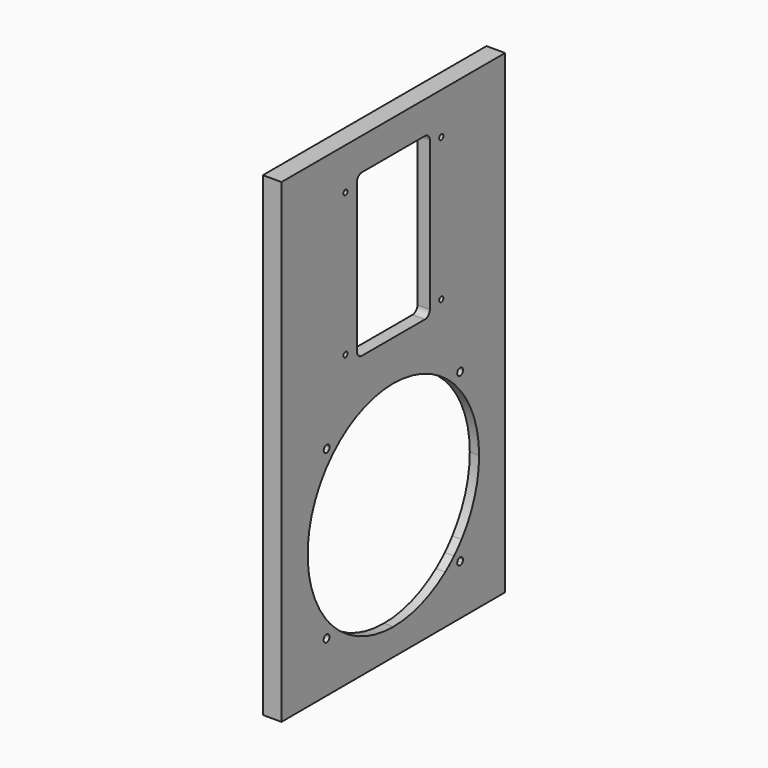
from build123d import *

# Parameters (mm, degrees)
F1_DEPTH = 9
F2_R     = 9
F3_DEPTH = 4.5
F4_DEPTH = 6


# Not quite as in the source:
# - ends of sketch curves that miss each other by under 0.0002 mm in the source are joined


with BuildPart() as f1:
    # F0 (on Right) → F1 (new body)
    with BuildSketch(Plane.YZ):
        Polygon((68.1698566968, 98.8894649375), (-66.8301433032, 98.8894649375), (-66.8301433032, -130.6578782697), (-12.3170643615, -130.5693798602), (0.7047325379, -130.5482398267), (13.9946170468, -130.5266645706), (68.1698566968, -130.438714621), align=None)
        with BuildLine():
            ThreePointArc((48.4358981994, -113.62957348), (25.065280219, -120.9302143017), (0.7053488138, -123.3957534174))
            ThreePointArc((0.7053488138, -123.3957534174), (-23.6541573557, -120.9260165144), (-47.0235169065, -113.6213484606))
            ThreePointArc((-47.0235169065, -113.6213484606), (-54.3241821931, -90.2506109118), (-56.7896968225, -65.8905549838))
            ThreePointArc((-56.7896968225, -65.8905549838), (-54.3199354552, -41.5311733414), (-47.015291887, -18.1619333547))
            ThreePointArc((-47.015291887, -18.1619333547), (-23.6446739066, -10.861292533), (0.7152574986, -8.3957534174))
            ThreePointArc((0.7152574986, -8.3957534174), (25.0747636681, -10.8654903203), (48.4441232188, -18.1701583742))
            ThreePointArc((48.4441232188, -18.1701583742), (58.2103031562, -65.9007077597), (48.4358981994, -113.62957348))
        make_face(mode=Mode.SUBTRACT)
        with BuildLine():
            add(Edge.make_bspline(
                [(29.3361078756, 2.5166290842), (19.796011102, -0.2153058112), (10.2559143284, -1.8939046488), (0.7158175548, -1.8957518912)],
                knots=[0.0757162728, 0.0757162728, 0.0757162728, 0.0757162728, 0.4997664403, 0.4997664403, 0.4997664403, 0.4997664403], degree=3))
            add(Edge.make_bspline(
                [(0.7158175548, -1.8957518912), (0.7105630297, -1.8957529086), (-8.8393481458, -1.8966775746), (-18.3892593212, -0.2170548711), (-27.9339159716, 2.5160323353)],
                knots=[0.4997664403, 0.4997664403, 0.4997664403, 0.4997664403, 0.5, 0.9242528506, 0.9242528506, 0.9242528506, 0.9242528506], degree=3))
            add(Edge.make_bspline(
                [(-27.9339159716, 2.5160323353), (-29.5600423042, 2.981669313), (-31.1861686369, 3.477911029), (-32.8122949696, 4.0016701601)],
                knots=[0.9242528506, 0.9242528506, 0.9242528506, 0.9242528506, 0.99653295, 0.99653295, 0.99653295, 0.99653295], degree=3))
            add(Edge.make_bspline(
                [(-32.8122949696, 4.0016701601), (-32.890295156, 4.026793245), (-32.9682953425, 4.0519796425), (-33.046295529, 4.0772290119)],
                knots=[0.99653295, 0.99653295, 0.99653295, 0.99653295, 1, 1, 1, 1], degree=3))
            add(Edge.make_bspline(
                [(-33.046295529, 4.0772290119), (-33.6603555303, 5.82974856), (-34.2037564934, 7.5898287802), (-34.6844360116, 9.3555033957)],
                knots=[0, 0, 0, 0, 0.0653643369, 0.0653643369, 0.0653643369, 0.0653643369], degree=3))
            add(Edge.make_bspline(
                [(-34.6844360116, 9.3555033957), (-37.9202250753, 21.2414906157), (-38.6995984681, 45.2840048827), (-37.8280446873, 67.9681639939), (-34.6344472565, 79.4497202748)],
                knots=[0.0653643369, 0.0653643369, 0.0653643369, 0.0653643369, 0.505377274, 0.9368183556, 0.9368183556, 0.9368183556, 0.9368183556], degree=3))
            add(Edge.make_bspline(
                [(-34.6344472565, 79.4497202748), (-34.166766394, 81.1311169635), (-33.6398504009, 82.8178973737), (-33.046295529, 84.5118955394)],
                knots=[0.9368183556, 0.9368183556, 0.9368183556, 0.9368183556, 1, 1, 1, 1], degree=3))
            add(Edge.make_bspline(
                [(-33.046295529, 84.5118955394), (-31.407102949, 85.0425170785), (-29.767910369, 85.5461701309), (-28.128717789, 86.0194468275)],
                knots=[0, 0, 0, 0, 0.0728608844, 0.0728608844, 0.0728608844, 0.0728608844], degree=3))
            add(Edge.make_bspline(
                [(-28.128717789, 86.0194468275), (-18.5191271995, 88.7939806713), (-8.9045783182, 90.52544354), (0.7099705632, 90.5245501515), (0.714928855, 90.5245492301)],
                knots=[0.0728608844, 0.0728608844, 0.0728608844, 0.0728608844, 0.5, 0.5002203924, 0.5002203924, 0.5002203924, 0.5002203924], degree=3))
            add(Edge.make_bspline(
                [(0.714928855, 90.5245492301), (10.3175892534, 90.5227648451), (19.9202496517, 88.7932594642), (29.52291005, 86.0211547084)],
                knots=[0.5002203924, 0.5002203924, 0.5002203924, 0.5002203924, 0.9270514662, 0.9270514662, 0.9270514662, 0.9270514662], degree=3))
            add(Edge.make_bspline(
                [(29.52291005, 86.0211547084), (31.1640745294, 85.5473818508), (32.8052390087, 85.0431554002), (34.4464034881, 84.5118955394)],
                knots=[0.9270514662, 0.9270514662, 0.9270514662, 0.9270514662, 1, 1, 1, 1], degree=3))
            add(Edge.make_bspline(
                [(34.4464034881, 84.5118955394), (35.0441587431, 82.8122899736), (35.5738699066, 81.1245502388), (36.0432502856, 79.4456408795)],
                knots=[0, 0, 0, 0, 0.0633907856, 0.0633907856, 0.0633907856, 0.0633907856], degree=3))
            add(Edge.make_bspline(
                [(36.0432502856, 79.4456408795), (39.2115398843, 68.1131027115), (40.0658474487, 45.8547250069), (39.3582763009, 21.3935099545), (36.0875285415, 9.3598851242)],
                knots=[0.0633907856, 0.0633907856, 0.0633907856, 0.0633907856, 0.4912748121, 0.9347375535, 0.9347375535, 0.9347375535, 0.9347375535], degree=3))
            add(Edge.make_bspline(
                [(36.0875285415, 9.3598851242), (35.6061870876, 7.5889498832), (35.0618079197, 5.8270167192), (34.4464034881, 4.0772290119)],
                knots=[0.9347375535, 0.9347375535, 0.9347375535, 0.9347375535, 1, 1, 1, 1], degree=3))
            add(Edge.make_bspline(
                [(34.4464034881, 4.0772290119), (34.3822403491, 4.0564588206), (34.3180772102, 4.0357312407), (34.2539140712, 4.015046462)],
                knots=[0, 0, 0, 0, 0.0028520035, 0.0028520035, 0.0028520035, 0.0028520035], degree=3))
            add(Edge.make_bspline(
                [(34.2539140712, 4.015046462), (32.6146453394, 3.4865824325), (30.9753766075, 2.9860557114), (29.3361078756, 2.5166290842)],
                knots=[0.0028520035, 0.0028520035, 0.0028520035, 0.0028520035, 0.0757162728, 0.0757162728, 0.0757162728, 0.0757162728], degree=3))
        make_face(mode=Mode.SUBTRACT)
        with BuildLine():
            ThreePointArc((33.489766199, 4.9329490876), (31.5635091045, 3.4659554383), (29.3361078756, 2.5166290842))
            add(Edge.make_bspline(
                [(34.2539140712, 4.015046462), (32.6146453394, 3.4865824325), (30.9753766075, 2.9860557114), (29.3361078756, 2.5166290842)],
                knots=[0.0028520035, 0.0028520035, 0.0028520035, 0.0028520035, 0.0757162728, 0.0757162728, 0.0757162728, 0.0757162728], degree=3))
            Line((34.2539140712, 4.015046462), (33.489766199, 4.9329490876))
        make_face()
        with BuildLine():
            add(Edge.make_bspline(
                [(-27.9339159716, 2.5160323353), (-29.5600423042, 2.981669313), (-31.1861686369, 3.477911029), (-32.8122949696, 4.0016701601)],
                knots=[0.9242528506, 0.9242528506, 0.9242528506, 0.9242528506, 0.99653295, 0.99653295, 0.99653295, 0.99653295], degree=3))
            ThreePointArc((-27.9339159716, 2.5160323353), (-30.1447439704, 3.4556982526), (-32.0601500824, 4.9055092414))
            Line((-32.0601500824, 4.9055092414), (-32.8122949696, 4.0016701601))
        make_face()
        with BuildLine():
            Line((33.489766199, 4.9329490876), (34.2539140712, 4.015046462))
            add(Edge.make_bspline(
                [(34.4464034881, 4.0772290119), (34.3822403491, 4.0564588206), (34.3180772102, 4.0357312407), (34.2539140712, 4.015046462)],
                knots=[0, 0, 0, 0, 0.0028520035, 0.0028520035, 0.0028520035, 0.0028520035], degree=3))
            add(Edge.make_bspline(
                [(36.0875285415, 9.3598851242), (35.6061870876, 7.5889498832), (35.0618079197, 5.8270167192), (34.4464034881, 4.0772290119)],
                knots=[0.9347375535, 0.9347375535, 0.9347375535, 0.9347375535, 1, 1, 1, 1], degree=3))
            ThreePointArc((36.0875285415, 9.3598851242), (35.0839686926, 6.9731201339), (33.489766199, 4.9329490876))
        make_face()
        with BuildLine():
            add(Edge.make_bspline(
                [(-32.8122949696, 4.0016701601), (-32.890295156, 4.026793245), (-32.9682953425, 4.0519796425), (-33.046295529, 4.0772290119)],
                knots=[0.99653295, 0.99653295, 0.99653295, 0.99653295, 1, 1, 1, 1], degree=3))
            Line((-32.8122949696, 4.0016701601), (-32.0601500824, 4.9055092414))
            ThreePointArc((-32.0601500824, 4.9055092414), (-33.6711503863, 6.9542617926), (-34.6844360116, 9.3555033957))
            add(Edge.make_bspline(
                [(-33.046295529, 4.0772290119), (-33.6603555303, 5.82974856), (-34.2037564934, 7.5898287802), (-34.6844360116, 9.3555033957)],
                knots=[0, 0, 0, 0, 0.0653643369, 0.0653643369, 0.0653643369, 0.0653643369], degree=3))
        make_face()
        with BuildLine():
            ThreePointArc((29.52291005, 86.0211547084), (33.6376071248, 83.5807546158), (36.0432502856, 79.4456408795))
            add(Edge.make_bspline(
                [(34.4464034881, 84.5118955394), (35.0441587431, 82.8122899736), (35.5738699066, 81.1245502388), (36.0432502856, 79.4456408795)],
                knots=[0, 0, 0, 0, 0.0633907856, 0.0633907856, 0.0633907856, 0.0633907856], degree=3))
            add(Edge.make_bspline(
                [(29.52291005, 86.0211547084), (31.1640745294, 85.5473818508), (32.8052390087, 85.0431554002), (34.4464034881, 84.5118955394)],
                knots=[0.9270514662, 0.9270514662, 0.9270514662, 0.9270514662, 1, 1, 1, 1], degree=3))
        make_face()
        with BuildLine():
            add(Edge.make_bspline(
                [(-34.6344472565, 79.4497202748), (-34.166766394, 81.1311169635), (-33.6398504009, 82.8178973737), (-33.046295529, 84.5118955394)],
                knots=[0.9368183556, 0.9368183556, 0.9368183556, 0.9368183556, 1, 1, 1, 1], degree=3))
            ThreePointArc((-34.6344472565, 79.4497202748), (-32.2364800237, 83.5811533161), (-28.128717789, 86.0194468275))
            add(Edge.make_bspline(
                [(-33.046295529, 84.5118955394), (-31.407102949, 85.0425170785), (-29.767910369, 85.5461701309), (-28.128717789, 86.0194468275)],
                knots=[0, 0, 0, 0, 0.0728608844, 0.0728608844, 0.0728608844, 0.0728608844], degree=3))
        make_face()
    extrude(amount=-F1_DEPTH)

    # F2
    f2_edges = [f1.edges().sort_by_distance(p)[0] for p in [
        (-4.5, 48.444123, -18.170158),
        (-4.5, -47.015292, -18.161933),
        (-4.5, 48.435898, -113.629573),
        (-4.5, -47.023517, -113.621348),
    ]]
    fillet(f2_edges, radius=F2_R)

    # F0 (on Right) → F3 (join)
    with BuildSketch(Plane.YZ):
        with BuildLine():
            ThreePointArc((-47.0235169065, -113.6213484606), (-23.6541573557, -120.9260165144), (0.7053488138, -123.3957534174))
            Line((0.7053488138, -123.3957534174), (0.7058442481, -117.6457532253))
            ThreePointArc((0.7058442481, -117.6457532253), (-15.8462466549, -114.9257764477), (-30.6588276682, -107.0544721939))
            ThreePointArc((-30.6588276682, -107.0544721939), (-37.7060174416, -114.9920661148), (-47.4126185448, -110.6966993112))
            ThreePointArc((-47.4126185448, -110.6966993112), (-48.2050884281, -108.8920718604), (-48.5857259237, -106.9582146141))
            add(Edge.make_bspline(
                [(-48.5857259237, -106.9582146141), (-52.8599458618, -93.2689444024), (-56.7908900644, -79.5796204898), (-56.7896968298, -65.8906363475), (-56.7896968225, -65.8905549838)],
                knots=[0.0417183372, 0.0417183372, 0.0417183372, 0.0417183372, 0.5000000605, 0.5000027845, 0.5000027845, 0.5000027845, 0.5000027845], degree=3))
            ThreePointArc((-56.7896968225, -65.8905549838), (-54.3241821931, -90.2506109118), (-47.0235169065, -113.6213484606))
        make_face()
        with BuildLine():
            Line((0.7058442481, -117.6457532253), (0.7053488138, -123.3957534174))
            ThreePointArc((0.7053488138, -123.3957534174), (25.065280219, -120.9302143017), (48.4358981994, -113.62957348))
            ThreePointArc((48.4358981994, -113.62957348), (58.2103031562, -65.9007077597), (48.4441232188, -18.1701583742))
            Line((48.4441232188, -18.1701583742), (42.246463418, -24.3667502557))
            ThreePointArc((42.246463418, -24.3667502557), (42.6184588324, -24.9309450129), (42.7489434931, -25.594021227))
            ThreePointArc((42.7489434931, -25.594021227), (41.6751090125, -27.2081154593), (39.7714575612, -26.8413296439))
            Line((39.7714575612, -26.8413296439), (37.3062318709, -29.3061305509))
            ThreePointArc((37.3062318709, -29.3061305509), (48.5219220944, -46.0939455578), (52.4603031562, -65.8957534174))
            ThreePointArc((52.4603031562, -65.8957534174), (49.7443824638, -82.4402862442), (41.8816918922, -97.2482533105))
            ThreePointArc((41.8816918922, -97.2482533105), (47.6632613149, -100.162881038), (49.9922390805, -106.2041940035))
            ThreePointArc((49.9922390805, -106.2041940035), (49.3222308171, -109.6117206236), (47.4119640434, -112.5118981342))
            ThreePointArc((47.4119640434, -112.5118981342), (37.9982171595, -114.6915865794), (32.0357152763, -107.0877557419))
            ThreePointArc((32.0357152763, -107.0877557419), (17.2365960025, -114.9359832777), (0.7058442481, -117.6457532253))
        make_face()
        with BuildLine():
            ThreePointArc((-47.4126185448, -110.6966993112), (-37.7060174416, -114.9920661148), (-30.6588276682, -107.0544721939))
            ThreePointArc((-30.6588276682, -107.0544721939), (-33.3488280366, -104.8577616098), (-35.8854305819, -102.4855712929))
            ThreePointArc((-35.8854305819, -102.4855712929), (-38.2656491214, -99.9389266546), (-40.4690269301, -97.2378221691))
            ThreePointArc((-40.4690269301, -97.2378221691), (-46.5261994153, -100.4289659711), (-48.5857259237, -106.9582146141))
            add(Edge.make_bspline(
                [(-47.4126185448, -110.6966993112), (-47.8046988201, -109.4505402503), (-48.1966348041, -108.2043773175), (-48.5857259237, -106.9582146141)],
                knots=[0, 0, 0, 0, 0.0417183372, 0.0417183372, 0.0417183372, 0.0417183372], degree=3))
        make_face()
        with BuildLine():
            ThreePointArc((-40.8454512075, -107.4447669293), (-40.8552676402, -104.9599498094), (-38.3704521876, -104.9701795704))
            ThreePointArc((-38.3704521876, -104.9701795704), (-37.9984287346, -105.5343880299), (-37.867933696, -106.1974895908))
            ThreePointArc((-37.867933696, -106.1974895908), (-38.9417886099, -107.8115923826), (-40.8454512075, -107.4447669293))
        make_face(mode=Mode.SUBTRACT)
        with BuildLine():
            ThreePointArc((37.3466484089, -102.4449080796), (34.7703842615, -104.8569312114), (32.0357152763, -107.0877557419))
            ThreePointArc((32.0357152763, -107.0877557419), (37.9982171595, -114.6915865794), (47.4119640434, -112.5118981342))
            Line((47.4119640434, -112.5118981342), (42.284825174, -107.3839063374))
            ThreePointArc((42.284825174, -107.3839063374), (39.754699299, -107.4415279477), (39.8127417737, -104.9114116926))
            Line((39.8127417737, -104.9114116926), (37.3466484089, -102.4449080796))
        make_face()
        with BuildLine():
            ThreePointArc((-47.015291887, -18.1619333547), (-54.3199354552, -41.5311733414), (-56.7896968225, -65.8905549838))
            add(Edge.make_bspline(
                [(-48.5857259237, -106.9582146141), (-52.8599458618, -93.2689444024), (-56.7908900644, -79.5796204898), (-56.7896968298, -65.8906363475), (-56.7896968225, -65.8905549838)],
                knots=[0.0417183372, 0.0417183372, 0.0417183372, 0.0417183372, 0.5000000605, 0.5000027845, 0.5000027845, 0.5000027845, 0.5000027845], degree=3))
            ThreePointArc((-48.5857259237, -106.9582146141), (-46.5261994153, -100.4289659711), (-40.4690269301, -97.2378221691))
            ThreePointArc((-40.4690269301, -97.2378221691), (-50.9220063581, -62.4076143407), (-35.8793197103, -29.2998247027))
            Line((-35.8793197103, -29.2998247027), (-38.353980194, -26.8247377365))
            ThreePointArc((-38.353980194, -26.8247377365), (-40.8288539189, -26.8245244952), (-40.8286406777, -24.3496507703))
            Line((-40.8286406777, -24.3496507703), (-45.9547231085, -19.2226849115))
            Line((-45.9547231085, -19.2226849115), (-47.015291887, -18.1619333547))
        make_face()
        with BuildLine():
            Line((42.246463418, -24.3667502557), (48.4441232188, -18.1701583742))
            ThreePointArc((48.4441232188, -18.1701583742), (25.0747636681, -10.8654903203), (0.7152574986, -8.3957534174))
            Line((0.7152574986, -8.3957534174), (0.7147620643, -14.1457536095))
            ThreePointArc((0.7147620643, -14.1457536095), (20.5182902015, -18.0866941376), (37.3062318709, -29.3061305509))
            Line((37.3062318709, -29.3061305509), (39.7714575612, -26.8413296439))
            ThreePointArc((39.7714575612, -26.8413296439), (39.7616132513, -24.3564777439), (42.246463418, -24.3667502557))
        make_face()
        with BuildLine():
            ThreePointArc((-48.5857259237, -106.9582146141), (-48.2050884281, -108.8920718604), (-47.4126185448, -110.6966993112))
            add(Edge.make_bspline(
                [(-47.4126185448, -110.6966993112), (-47.8046988201, -109.4505402503), (-48.1966348041, -108.2043773175), (-48.5857259237, -106.9582146141)],
                knots=[0, 0, 0, 0, 0.0417183372, 0.0417183372, 0.0417183372, 0.0417183372], degree=3))
        make_face()
        with BuildLine():
            ThreePointArc((41.8816918922, -97.2482533105), (39.7008426794, -99.9222185246), (37.3466484089, -102.4449080796))
            Line((37.3466484089, -102.4449080796), (39.8127417737, -104.9114116926))
            ThreePointArc((39.8127417737, -104.9114116926), (41.6987727715, -104.6031599179), (42.7422390805, -106.2041940035))
            ThreePointArc((42.7422390805, -106.2041940035), (42.6238832916, -106.8368370056), (42.284825174, -107.3839063374))
            Line((42.284825174, -107.3839063374), (47.4119640434, -112.5118981342))
            ThreePointArc((47.4119640434, -112.5118981342), (49.3222308171, -109.6117206236), (49.9922390805, -106.2041940035))
            ThreePointArc((49.9922390805, -106.2041940035), (47.6632613149, -100.162881038), (41.8816918922, -97.2482533105))
        make_face()
        with BuildLine():
            ThreePointArc((0.7152574986, -8.3957534174), (-23.6446739066, -10.861292533), (-47.015291887, -18.1619333547))
            Line((-47.015291887, -18.1619333547), (-45.9547231085, -19.2226849115))
            Line((-45.9547231085, -19.2226849115), (-40.8286406777, -24.3496507703))
            ThreePointArc((-40.8286406777, -24.3496507703), (-38.9215447765, -23.9704339243), (-37.8413104358, -25.5871942534))
            ThreePointArc((-37.8413104358, -25.5871942534), (-37.9745501068, -26.2569599127), (-38.353980194, -26.8247377365))
            Line((-38.353980194, -26.8247377365), (-35.8793197103, -29.2998247027))
            ThreePointArc((-35.8793197103, -29.2998247027), (-19.0894449013, -18.0832814371), (0.7147620643, -14.1457536095))
            Line((0.7147620643, -14.1457536095), (0.7152574986, -8.3957534174))
        make_face()
        with BuildLine():
            ThreePointArc((33.489766199, 4.9329490876), (31.5635091045, 3.4659554383), (29.3361078756, 2.5166290842))
            add(Edge.make_bspline(
                [(34.2539140712, 4.015046462), (32.6146453394, 3.4865824325), (30.9753766075, 2.9860557114), (29.3361078756, 2.5166290842)],
                knots=[0.0028520035, 0.0028520035, 0.0028520035, 0.0028520035, 0.0757162728, 0.0757162728, 0.0757162728, 0.0757162728], degree=3))
            Line((34.2539140712, 4.015046462), (33.489766199, 4.9329490876))
        make_face()
        with BuildLine():
            add(Edge.make_bspline(
                [(-27.9339159716, 2.5160323353), (-29.5600423042, 2.981669313), (-31.1861686369, 3.477911029), (-32.8122949696, 4.0016701601)],
                knots=[0.9242528506, 0.9242528506, 0.9242528506, 0.9242528506, 0.99653295, 0.99653295, 0.99653295, 0.99653295], degree=3))
            ThreePointArc((-27.9339159716, 2.5160323353), (-30.1447439704, 3.4556982526), (-32.0601500824, 4.9055092414))
            Line((-32.0601500824, 4.9055092414), (-32.8122949696, 4.0016701601))
        make_face()
        with BuildLine():
            Line((33.489766199, 4.9329490876), (34.2539140712, 4.015046462))
            add(Edge.make_bspline(
                [(34.4464034881, 4.0772290119), (34.3822403491, 4.0564588206), (34.3180772102, 4.0357312407), (34.2539140712, 4.015046462)],
                knots=[0, 0, 0, 0, 0.0028520035, 0.0028520035, 0.0028520035, 0.0028520035], degree=3))
            add(Edge.make_bspline(
                [(36.0875285415, 9.3598851242), (35.6061870876, 7.5889498832), (35.0618079197, 5.8270167192), (34.4464034881, 4.0772290119)],
                knots=[0.9347375535, 0.9347375535, 0.9347375535, 0.9347375535, 1, 1, 1, 1], degree=3))
            ThreePointArc((36.0875285415, 9.3598851242), (35.0839686926, 6.9731201339), (33.489766199, 4.9329490876))
        make_face()
        with BuildLine():
            Line((30.2969391288, 8.7682072326), (33.489766199, 4.9329490876))
            ThreePointArc((33.489766199, 4.9329490876), (35.0839686926, 6.9731201339), (36.0875285415, 9.3598851242))
            add(Edge.make_bspline(
                [(36.0432502856, 79.4456408795), (39.2115398843, 68.1131027115), (40.0658474487, 45.8547250069), (39.3582763009, 21.3935099545), (36.0875285415, 9.3598851242)],
                knots=[0.0633907856, 0.0633907856, 0.0633907856, 0.0633907856, 0.4912748121, 0.9347375535, 0.9347375535, 0.9347375535, 0.9347375535], degree=3))
            ThreePointArc((36.0432502856, 79.4456408795), (33.6376071248, 83.5807546158), (29.52291005, 86.0211547084))
            add(Edge.make_bspline(
                [(0.714928855, 90.5245492301), (10.3175892534, 90.5227648451), (19.9202496517, 88.7932594642), (29.52291005, 86.0211547084)],
                knots=[0.5002203924, 0.5002203924, 0.5002203924, 0.5002203924, 0.9270514662, 0.9270514662, 0.9270514662, 0.9270514662], degree=3))
            Line((0.714928855, 90.5245492301), (0.7156901067, 83.2965870832))
            Line((0.7156901067, 83.2965870832), (19.7197976011, 83.2965870832))
            ThreePointArc((19.7197976011, 83.2965870832), (21.8411179447, 82.4179074268), (22.7197976011, 80.2965870832))
            Line((22.7197976011, 80.2965870832), (22.7197976011, 78.7713235))
            Line((22.7197976011, 78.7713235), (22.7197976011, 17.8699509601))
            Line((22.7197976011, 17.8699509601), (28.7103497083, 10.6740354731))
            ThreePointArc((28.7103497083, 10.6740354731), (30.0829713415, 10.9858407594), (30.8754964154, 9.8225623353))
            ThreePointArc((30.8754964154, 9.8225623353), (30.7213530191, 9.2212318902), (30.2969391288, 8.7682072326))
        make_face()
        with BuildLine():
            ThreePointArc((30.87627166, 78.7719689719), (29.6263300718, 77.5219689733), (28.3762716654, 78.7718521482))
            ThreePointArc((28.3762716654, 78.7718521482), (29.6262132481, 80.0219689705), (30.87627166, 78.7719689719))
        make_face(mode=Mode.SUBTRACT)
        with BuildLine():
            add(Edge.make_bspline(
                [(-32.8122949696, 4.0016701601), (-32.890295156, 4.026793245), (-32.9682953425, 4.0519796425), (-33.046295529, 4.0772290119)],
                knots=[0.99653295, 0.99653295, 0.99653295, 0.99653295, 1, 1, 1, 1], degree=3))
            Line((-32.8122949696, 4.0016701601), (-32.0601500824, 4.9055092414))
            ThreePointArc((-32.0601500824, 4.9055092414), (-33.6711503863, 6.9542617926), (-34.6844360116, 9.3555033957))
            add(Edge.make_bspline(
                [(-33.046295529, 4.0772290119), (-33.6603555303, 5.82974856), (-34.2037564934, 7.5898287802), (-34.6844360116, 9.3555033957)],
                knots=[0, 0, 0, 0, 0.0653643369, 0.0653643369, 0.0653643369, 0.0653643369], degree=3))
        make_face()
        with BuildLine():
            ThreePointArc((-34.6844360116, 9.3555033957), (-33.6711503863, 6.9542617926), (-32.0601500824, 4.9055092414))
            Line((-32.0601500824, 4.9055092414), (-28.8630317223, 8.7474292898))
            ThreePointArc((-28.8630317223, 8.7474292898), (-29.1862160537, 10.6221311742), (-27.2839974447, 10.6449265874))
            Line((-27.2839974447, 10.6449265874), (-21.2802023989, 17.8595798955))
            Line((-21.2802023989, 17.8595798955), (-21.2802023989, 78.7672113059))
            Line((-21.2802023989, 78.7672113059), (-21.2802023989, 80.2965870832))
            ThreePointArc((-21.2802023989, 80.2965870832), (-20.4015227424, 82.4179074268), (-18.2802023989, 83.2965870832))
            Line((-18.2802023989, 83.2965870832), (0.7156901067, 83.2965870832))
            Line((0.7156901067, 83.2965870832), (0.714928855, 90.5245492301))
            add(Edge.make_bspline(
                [(-28.128717789, 86.0194468275), (-18.5191271995, 88.7939806713), (-8.9045783182, 90.52544354), (0.7099705632, 90.5245501515), (0.714928855, 90.5245492301)],
                knots=[0.0728608844, 0.0728608844, 0.0728608844, 0.0728608844, 0.5, 0.5002203924, 0.5002203924, 0.5002203924, 0.5002203924], degree=3))
            ThreePointArc((-28.128717789, 86.0194468275), (-32.2364800237, 83.5811533161), (-34.6344472565, 79.4497202748))
            add(Edge.make_bspline(
                [(-34.6844360116, 9.3555033957), (-37.9202250753, 21.2414906157), (-38.6995984681, 45.2840048827), (-37.8280446873, 67.9681639939), (-34.6344472565, 79.4497202748)],
                knots=[0.0653643369, 0.0653643369, 0.0653643369, 0.0653643369, 0.505377274, 0.9368183556, 0.9368183556, 0.9368183556, 0.9368183556], degree=3))
        make_face()
        with BuildLine():
            ThreePointArc((-26.9753884564, 78.766562216), (-29.475388455, 78.7665038042), (-26.9753884618, 78.7666790397))
            ThreePointArc((-26.9753884618, 78.7666790397), (-26.9753884577, 78.7666206279), (-26.9753884564, 78.766562216))
        make_face(mode=Mode.SUBTRACT)
        with BuildLine():
            ThreePointArc((29.52291005, 86.0211547084), (33.6376071248, 83.5807546158), (36.0432502856, 79.4456408795))
            add(Edge.make_bspline(
                [(34.4464034881, 84.5118955394), (35.0441587431, 82.8122899736), (35.5738699066, 81.1245502388), (36.0432502856, 79.4456408795)],
                knots=[0, 0, 0, 0, 0.0633907856, 0.0633907856, 0.0633907856, 0.0633907856], degree=3))
            add(Edge.make_bspline(
                [(29.52291005, 86.0211547084), (31.1640745294, 85.5473818508), (32.8052390087, 85.0431554002), (34.4464034881, 84.5118955394)],
                knots=[0.9270514662, 0.9270514662, 0.9270514662, 0.9270514662, 1, 1, 1, 1], degree=3))
        make_face()
        with BuildLine():
            add(Edge.make_bspline(
                [(-34.6344472565, 79.4497202748), (-34.166766394, 81.1311169635), (-33.6398504009, 82.8178973737), (-33.046295529, 84.5118955394)],
                knots=[0.9368183556, 0.9368183556, 0.9368183556, 0.9368183556, 1, 1, 1, 1], degree=3))
            ThreePointArc((-34.6344472565, 79.4497202748), (-32.2364800237, 83.5811533161), (-28.128717789, 86.0194468275))
            add(Edge.make_bspline(
                [(-33.046295529, 84.5118955394), (-31.407102949, 85.0425170785), (-29.767910369, 85.5461701309), (-28.128717789, 86.0194468275)],
                knots=[0, 0, 0, 0, 0.0728608844, 0.0728608844, 0.0728608844, 0.0728608844], degree=3))
        make_face()
    extrude(amount=-F3_DEPTH)

    # F0 (on Right) → F4 (join)
    with BuildSketch(Plane.YZ):
        with BuildLine():
            Line((30.2969391288, 8.7682072326), (33.489766199, 4.9329490876))
            ThreePointArc((33.489766199, 4.9329490876), (35.0839686926, 6.9731201339), (36.0875285415, 9.3598851242))
            add(Edge.make_bspline(
                [(36.0432502856, 79.4456408795), (39.2115398843, 68.1131027115), (40.0658474487, 45.8547250069), (39.3582763009, 21.3935099545), (36.0875285415, 9.3598851242)],
                knots=[0.0633907856, 0.0633907856, 0.0633907856, 0.0633907856, 0.4912748121, 0.9347375535, 0.9347375535, 0.9347375535, 0.9347375535], degree=3))
            ThreePointArc((36.0432502856, 79.4456408795), (33.6376071248, 83.5807546158), (29.52291005, 86.0211547084))
            add(Edge.make_bspline(
                [(0.714928855, 90.5245492301), (10.3175892534, 90.5227648451), (19.9202496517, 88.7932594642), (29.52291005, 86.0211547084)],
                knots=[0.5002203924, 0.5002203924, 0.5002203924, 0.5002203924, 0.9270514662, 0.9270514662, 0.9270514662, 0.9270514662], degree=3))
            Line((0.714928855, 90.5245492301), (0.7156901067, 83.2965870832))
            Line((0.7156901067, 83.2965870832), (19.7197976011, 83.2965870832))
            ThreePointArc((19.7197976011, 83.2965870832), (21.8411179447, 82.4179074268), (22.7197976011, 80.2965870832))
            Line((22.7197976011, 80.2965870832), (22.7197976011, 78.7713235))
            Line((22.7197976011, 78.7713235), (22.7197976011, 17.8699509601))
            Line((22.7197976011, 17.8699509601), (28.7103497083, 10.6740354731))
            ThreePointArc((28.7103497083, 10.6740354731), (30.0829713415, 10.9858407594), (30.8754964154, 9.8225623353))
            ThreePointArc((30.8754964154, 9.8225623353), (30.7213530191, 9.2212318902), (30.2969391288, 8.7682072326))
        make_face()
        with BuildLine():
            ThreePointArc((30.87627166, 78.7719689719), (29.6263300718, 77.5219689733), (28.3762716654, 78.7718521482))
            ThreePointArc((28.3762716654, 78.7718521482), (29.6262132481, 80.0219689705), (30.87627166, 78.7719689719))
        make_face(mode=Mode.SUBTRACT)
        with BuildLine():
            ThreePointArc((-34.6844360116, 9.3555033957), (-33.6711503863, 6.9542617926), (-32.0601500824, 4.9055092414))
            Line((-32.0601500824, 4.9055092414), (-28.8630317223, 8.7474292898))
            ThreePointArc((-28.8630317223, 8.7474292898), (-29.1862160537, 10.6221311742), (-27.2839974447, 10.6449265874))
            Line((-27.2839974447, 10.6449265874), (-21.2802023989, 17.8595798955))
            Line((-21.2802023989, 17.8595798955), (-21.2802023989, 78.7672113059))
            Line((-21.2802023989, 78.7672113059), (-21.2802023989, 80.2965870832))
            ThreePointArc((-21.2802023989, 80.2965870832), (-20.4015227424, 82.4179074268), (-18.2802023989, 83.2965870832))
            Line((-18.2802023989, 83.2965870832), (0.7156901067, 83.2965870832))
            Line((0.7156901067, 83.2965870832), (0.714928855, 90.5245492301))
            add(Edge.make_bspline(
                [(-28.128717789, 86.0194468275), (-18.5191271995, 88.7939806713), (-8.9045783182, 90.52544354), (0.7099705632, 90.5245501515), (0.714928855, 90.5245492301)],
                knots=[0.0728608844, 0.0728608844, 0.0728608844, 0.0728608844, 0.5, 0.5002203924, 0.5002203924, 0.5002203924, 0.5002203924], degree=3))
            ThreePointArc((-28.128717789, 86.0194468275), (-32.2364800237, 83.5811533161), (-34.6344472565, 79.4497202748))
            add(Edge.make_bspline(
                [(-34.6844360116, 9.3555033957), (-37.9202250753, 21.2414906157), (-38.6995984681, 45.2840048827), (-37.8280446873, 67.9681639939), (-34.6344472565, 79.4497202748)],
                knots=[0.0653643369, 0.0653643369, 0.0653643369, 0.0653643369, 0.505377274, 0.9368183556, 0.9368183556, 0.9368183556, 0.9368183556], degree=3))
        make_face()
        with BuildLine():
            ThreePointArc((-26.9753884564, 78.766562216), (-29.475388455, 78.7665038042), (-26.9753884618, 78.7666790397))
            ThreePointArc((-26.9753884618, 78.7666790397), (-26.9753884577, 78.7666206279), (-26.9753884564, 78.766562216))
        make_face(mode=Mode.SUBTRACT)
        with BuildLine():
            Line((0.7164372645, 5.2965870832), (0.7158175548, -1.8957518912))
            add(Edge.make_bspline(
                [(29.3361078756, 2.5166290842), (19.796011102, -0.2153058112), (10.2559143284, -1.8939046488), (0.7158175548, -1.8957518912)],
                knots=[0.0757162728, 0.0757162728, 0.0757162728, 0.0757162728, 0.4997664403, 0.4997664403, 0.4997664403, 0.4997664403], degree=3))
            ThreePointArc((29.3361078756, 2.5166290842), (31.5635091045, 3.4659554383), (33.489766199, 4.9329490876))
            Line((33.489766199, 4.9329490876), (30.2969391288, 8.7682072326))
            ThreePointArc((30.2969391288, 8.7682072326), (28.6648230944, 9.0228081417), (28.7103497083, 10.6740354731))
            Line((28.7103497083, 10.6740354731), (22.7197976011, 17.8699509601))
            Line((22.7197976011, 17.8699509601), (22.7197976011, 8.2965870832))
            ThreePointArc((22.7197976011, 8.2965870832), (21.8411179447, 6.1752667396), (19.7197976011, 5.2965870832))
            Line((19.7197976011, 5.2965870832), (0.7164372645, 5.2965870832))
        make_face()
        with BuildLine():
            add(Edge.make_bspline(
                [(0.7158175548, -1.8957518912), (0.7105630297, -1.8957529086), (-8.8393481458, -1.8966775746), (-18.3892593212, -0.2170548711), (-27.9339159716, 2.5160323353)],
                knots=[0.4997664403, 0.4997664403, 0.4997664403, 0.4997664403, 0.5, 0.9242528506, 0.9242528506, 0.9242528506, 0.9242528506], degree=3))
            Line((0.7158175548, -1.8957518912), (0.7164372645, 5.2965870832))
            Line((0.7164372645, 5.2965870832), (-18.2802023989, 5.2965870832))
            ThreePointArc((-18.2802023989, 5.2965870832), (-20.4015227424, 6.1752667396), (-21.2802023989, 8.2965870832))
            Line((-21.2802023989, 8.2965870832), (-21.2802023989, 17.8595798955))
            Line((-21.2802023989, 17.8595798955), (-27.2839974447, 10.6449265874))
            ThreePointArc((-27.2839974447, 10.6449265874), (-27.0550810684, 10.2617440946), (-26.9753884564, 9.8225623353))
            ThreePointArc((-26.9753884564, 9.8225623353), (-27.6067423873, 8.7363869161), (-28.8630317223, 8.7474292898))
            Line((-28.8630317223, 8.7474292898), (-32.0601500824, 4.9055092414))
            ThreePointArc((-32.0601500824, 4.9055092414), (-30.1447439704, 3.4556982526), (-27.9339159716, 2.5160323353))
        make_face()
    extrude(amount=-F4_DEPTH)


solid = f1.part
